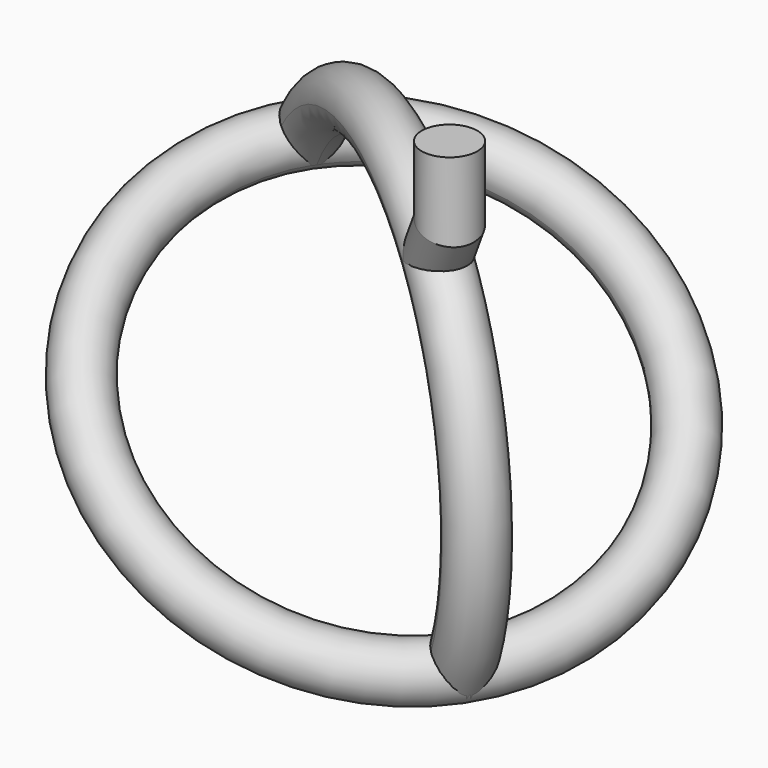
from build123d import *

# Parameters (mm, degrees)
F3_R     = 25
F7_ANGLE = 213.75


with BuildPart() as f4:
    # F4: sweep along a path in F0
    with BuildLine(Plane.XZ) as f4_path:
        Line((0, 0), (0, -63.5))
        Line((0, -63.5), (28.9665412822, -104.8685081943))
    # F3 (on Top) → F4 (sweep)
    with BuildSketch(Plane.XY):
        Circle(F3_R)
    sweep(path=f4_path.line, transition=Transition.RIGHT)


with BuildPart() as f5:
    # F5: sweep along a path in F0
    with BuildLine(Plane.XZ) as f5_path:
        ThreePointArc((329.0286556186, -157.6999922858), (28.9665412822, -104.8685081943), (-24.0153903238, -404.9040945747))
    # F2 (on face) → F5 (sweep)
    with BuildSketch(Plane(origin=(182.3418733573, 0, -260.4111829809), x_dir=(0.8191520443, 0, 0.5735764364), z_dir=(0.5735764364, 0, -0.8191520443))):
        with BuildLine():
            ThreePointArc((-250.2837609958, -24.9574575102), (-251.7416068816, 0), (-250.2991347517, 24.95835079))
            ThreePointArc((-250.2991347517, 24.95835079), (-276.7416056959, -0.0076998428), (-250.2837609958, -24.9574575102))
        make_face()
        with BuildLine():
            ThreePointArc((-226.7416068816, 0), (-233.5610980432, 17.1601019337), (-250.2991347517, 24.95835079))
            ThreePointArc((-250.2991347517, 24.95835079), (-251.7416068816, 0), (-250.2837609958, -24.9574575102))
            ThreePointArc((-250.2837609958, -24.9574575102), (-233.555813702, -17.1545016374), (-226.7416068816, 0))
        make_face()
    sweep(path=f5_path.line)


with BuildPart() as f6:
    # F6: sweep along a path in F2
    with BuildLine(Plane(origin=(182.3418733573, 0, -260.4111829809), x_dir=(0.8191520443, 0, 0.5735764364), z_dir=(0.5735764364, 0, -0.8191520443))) as f6_path:
        CenterArc((-36.2480171025, 0.0663706742), 215.4936, 0, 360)
    # F0 (on Front) → F6 (sweep)
    with BuildSketch(Plane.XZ):
        with BuildLine():
            ThreePointArc((0.9846096762, -404.9040945747), (-0.1724665551, -397.3864495871), (-3.5365892166, -390.564683666))
            Line((-3.5365892166, -390.564683666), (-24.0153903238, -404.9040945747))
            ThreePointArc((-24.0153903238, -404.9040945747), (-30.8826310352, -394.4531299469), (-37.1320864089, -383.6214189015))
            ThreePointArc((-37.1320864089, -383.6214189015), (-36.2031423289, -426.732028537), (0.9846096762, -404.9040945747))
        make_face()
        with BuildLine():
            Line((-24.0153903238, -404.9040945747), (-3.5365892166, -390.564683666))
            ThreePointArc((-3.5365892166, -390.564683666), (-18.9555109788, -380.4214962442), (-37.1320864089, -383.6214189015))
            ThreePointArc((-37.1320864089, -383.6214189015), (-30.8826310352, -394.4531299469), (-24.0153903238, -404.9040945747))
        make_face()
    sweep(path=f6_path.line)


with BuildPart() as f5_1:
    # F7: moved
    add(f5.part.rotate(Axis((0, 0, -31.75), (0, 0, -1)), F7_ANGLE))


with BuildPart() as f6_1:
    # F7: moved
    add(f6.part.rotate(Axis((0, 0, -31.75), (0, 0, -1)), F7_ANGLE))


with BuildPart() as f4_1:
    # F7: moved
    add(f4.part.rotate(Axis((0, 0, -31.75), (0, 0, -1)), F7_ANGLE))


solid = Compound([f5_1.part, f6_1.part, f4_1.part])
